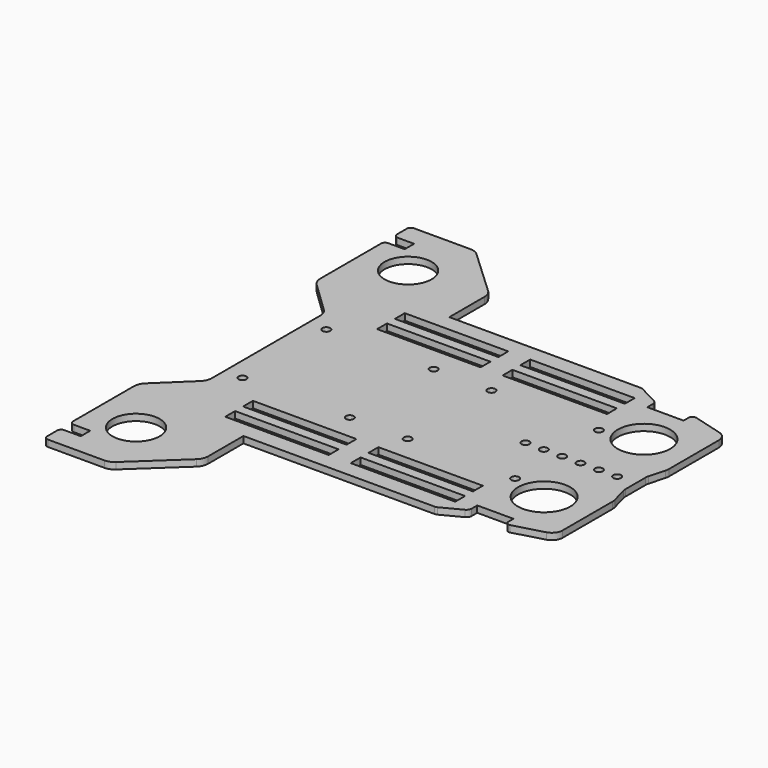
from build123d import *
from build123d import SkipClean  # not in build123d's __all__

# Parameters (mm, degrees)
F0_R      = 9
F0_W      = 39.5156368613
F0_H      = 4.7
F0_W_2    = 39.887715684
F0_R_2    = 10
F1_DEPTH  = 2.5
F2_R      = 1.4160019586
F3_R      = 4.1166770091
F4_R      = 2.0561745665
F5_R      = 5
F6_R      = 1.5425858978
F7_R      = 5
F8_R      = 5
F10_R     = 1.5
F11_DEPTH = 25


with BuildPart() as f1:
    # F0 (on Top) → F1 (new body)
    with BuildSketch(Plane.XY):
        with BuildLine():
            Line((74.8763903975, -38.2511245025), (69.3773250177, -38.2511245025))
            ThreePointArc((69.3773250177, -38.2511245025), (67.8773250177, -39.7511245025), (66.3773250177, -38.2511245025))
            Line((66.3773250177, -38.2511245025), (62.3773250177, -38.2511245025))
            ThreePointArc((62.3773250177, -38.2511245025), (60.8773250177, -39.7511245025), (59.3773250177, -38.2511245025))
            Line((59.3773250177, -38.2511245025), (55.3773250177, -38.2511245025))
            ThreePointArc((55.3773250177, -38.2511245025), (53.8773250177, -39.7511245025), (52.3773250177, -38.2511245025))
            Line((52.3773250177, -38.2511245025), (48.3773250177, -38.2511245025))
            ThreePointArc((48.3773250177, -38.2511245025), (46.8773250177, -39.7511245025), (45.3773250177, -38.2511245025))
            Line((45.3773250177, -38.2511245025), (41.3773250177, -38.2511245025))
            ThreePointArc((41.3773250177, -38.2511245025), (39.8773250177, -39.7511245025), (38.3773250177, -38.2511245025))
            Line((38.3773250177, -38.2511245025), (34.3773250177, -38.2511245025))
            ThreePointArc((34.3773250177, -38.2511245025), (32.8773250177, -39.7511245025), (31.3773250177, -38.2511245025))
            Line((31.3773250177, -38.2511245025), (-66.1923438311, -38.2511245025))
            Line((-66.1923438311, -38.2511245025), (-66.1923438311, -66.2511245025))
            Line((-66.1923438311, -66.2511245025), (-81.1216448216, -80.6109128623))
            Line((-81.1216448216, -80.6109128623), (-81.1216448216, -113.3109128623))
            Line((-81.1216448216, -113.3109128623), (-73.3216448216, -113.3109128623))
            Line((-73.3216448216, -113.3109128623), (-73.3216448216, -117.8109128623))
            Line((-73.3216448216, -117.8109128623), (-81.1216448216, -117.8109128623))
            Line((-81.1216448216, -117.8109128623), (-81.1216448216, -125.6109128623))
            Line((-81.1216448216, -125.6109128623), (-56.1216448216, -125.6109128623))
            Line((-56.1216448216, -125.6109128623), (-35.532054749, -106.3894852996))
            Line((-35.532054749, -106.3894852996), (-35.532054749, -87.3894852996))
            Line((-35.532054749, -87.3894852996), (38.0006051308, -87.3894852996))
            Line((38.0006051308, -87.3894852996), (46.9109937549, -82.7472803621))
            Line((46.9109937549, -82.7472803621), (46.9109937549, -78.8513062))
            Line((46.9109937549, -78.8513062), (60.7595592737, -78.8513062))
            Line((60.7595592737, -78.8513062), (60.7595592737, -83.155875459))
            Line((60.7595592737, -83.155875459), (76.8783551784, -78.677393496))
            Line((76.8783551784, -78.677393496), (76.8783551784, -51.0392449796))
            Line((76.8783551784, -51.0392449796), (74.8763903975, -43.6687730253))
            Line((74.8763903975, -43.6687730253), (74.8763903975, -38.2511245025))
        make_face()
        with Locations((-63.9078766108, -103.1785532832)):
            Circle(F0_R, mode=Mode.SUBTRACT)
        with Locations((-27.756717056, -78.7394852996)):
            Rectangle(F0_W, F0_H, mode=Mode.SUBTRACT)
        with Locations((-27.756717056, -70.2394852996)):
            Rectangle(F0_W, F0_H, mode=Mode.SUBTRACT)
        with Locations((20.3393899865, -78.7394852996)):
            Rectangle(F0_W_2, F0_H, mode=Mode.SUBTRACT)
        with Locations((20.3393899865, -70.2394852996)):
            Rectangle(F0_W_2, F0_H, mode=Mode.SUBTRACT)
        with Locations((59.0378009468, -62.0803784949)):
            Circle(F0_R_2, mode=Mode.SUBTRACT)
    extrude(amount=F1_DEPTH)

    # F2
    f2_edges = [f1.edges().sort_by_distance(p)[0] for p in [
        (60.759559, -83.155875, 1.25),
    ]]
    fillet(f2_edges, radius=F2_R)

    # F3
    f3_edges = [f1.edges().sort_by_distance(p)[0] for p in [
        (76.878355, -78.677393, 1.25),
    ]]
    fillet(f3_edges, radius=F3_R)

    # F4
    f4_edges = [f1.edges().sort_by_distance(p)[0] for p in [
        (46.910994, -82.74728, 1.25),
        (38.000605, -87.389485, 1.25),
    ]]
    fillet(f4_edges, radius=F4_R)

    # F5
    f5_edges = [f1.edges().sort_by_distance(p)[0] for p in [
        (-56.121645, -125.610913, 1.25),
        (-35.532055, -106.389485, 1.25),
    ]]
    fillet(f5_edges, radius=F5_R)

    # F6
    f6_edges = [f1.edges().sort_by_distance(p)[0] for p in [
        (-81.121645, -113.310913, 1.25),
        (-81.121645, -117.810913, 1.25),
        (-81.121645, -125.610913, 1.25),
    ]]
    fillet(f6_edges, radius=F6_R)

    # F7
    f7_edges = [f1.edges().sort_by_distance(p)[0] for p in [
        (-81.121645, -80.610913, 1.25),
        (-66.192344, -66.251125, 1.25),
    ]]
    fillet(f7_edges, radius=F7_R)

    # F8
    f8_edges = [f1.edges().sort_by_distance(p)[0] for p in [
        (76.878355, -51.039245, 1.25),
        (74.87639, -43.668773, 1.25),
    ]]
    fillet(f8_edges, radius=F8_R)

    # F9: F1 across face


with BuildPart() as f1_1:
    add(f1.part, clean=False)
    with SkipClean():  # cleaning this boolean's faces spoils the solid; the shape is the same uncleaned
        add(f1.part.mirror(Plane(origin=(-17.4075094067, -38.2511245025, 1.25), x_dir=(-1, 0, 0), z_dir=(0, 1, 0))), clean=False)

    # F10 (on face) → F11 (cut)
    with BuildSketch(Plane.XY.offset(2.5)):
        with Locations((-59.1923438311, -18.2511245025)):
            Circle(F10_R)
        with Locations((-18.1923438311, -18.2511245025)):
            Circle(F10_R)
        with Locations((-18.1923438311, -58.2511245025)):
            Circle(F10_R)
        with Locations((-59.1923438311, -58.2511245025)):
            Circle(F10_R)
        with Locations((3.8763903975, -18.2511245025)):
            Circle(F10_R)
        with Locations((3.8763903975, -58.2511245025)):
            Circle(F10_R)
        with Locations((44.8763903975, -58.2511245025)):
            Circle(F10_R)
        with Locations((44.8763903975, -18.2511245025)):
            Circle(F10_R)
    extrude(amount=-F11_DEPTH, mode=Mode.SUBTRACT)


solid = f1_1.part
